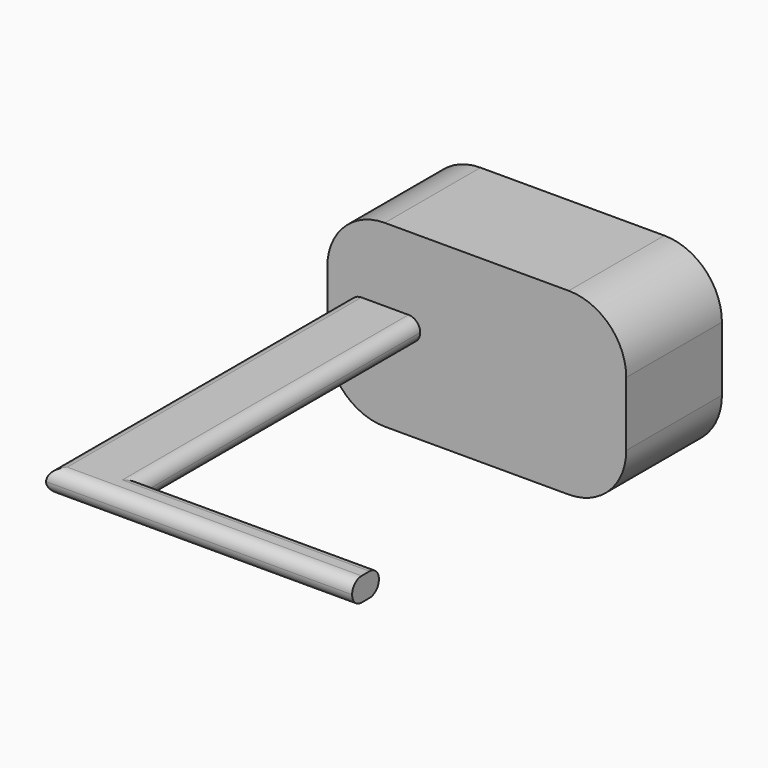
from build123d import *

# Parameters (mm, degrees)
F0_W     = 127
F0_H     = 76.2
F1_DEPTH = 50.8
F2_R     = 24.4421069165
F4_W     = 30
F4_H     = 10
F5_DEPTH = 211.9498550892
F6_W     = 14.2212212086
F6_H     = 10
F7_DEPTH = 100
F8_R     = 4.99999


# Not quite as in the source:
# - a fillet or chamfer is up to 0.001 mm smaller than in the source, because OpenCascade refuses the exact size


with BuildPart() as f1:
    # F0 (on Front) → F1 (new body)
    with BuildSketch(Plane.XZ):
        with Locations((21.6533541679, 32.7783897177)):
            Rectangle(F0_W, F0_H)
    extrude(amount=F1_DEPTH)

    # F2
    f2_edges = [f1.edges().sort_by_distance(p)[0] for p in [
        (-41.846646, -25.4, 70.87839),
        (-41.846646, -25.4, -5.32161),
        (85.153354, -25.4, -5.32161),
        (85.153354, -25.4, 70.87839),
    ]]
    fillet(f2_edges, radius=F2_R)

    # F4 (on face) → F5 (join)
    with BuildSketch(Plane(origin=(0, 0, 0), x_dir=(-1, 0, 0), z_dir=(0, 1, 0))):
        with Locations((17.3587081618, 34.757822752)):
            Rectangle(F4_W, F4_H)
    extrude(amount=-F5_DEPTH)

    # F6 (on face) → F7 (join)
    with BuildSketch(Plane.YZ.offset(-2.3587081618)):
        with Locations((-204.8392444849, 34.757822752)):
            Rectangle(F6_W, F6_H)
    extrude(amount=F7_DEPTH)

    # F8 (radius 5 in the source; OpenCascade refuses exactly that, so slightly less here)
    f8_edges = [f1.edges().sort_by_distance(p)[0] for p in [
        (-32.358708, -131.374928, 39.757823),
        (-32.358708, -131.374928, 29.757823),
        (32.641292, -211.949855, 29.757823),
        (-2.358708, -124.264317, 29.757823),
        (-2.358708, -124.264317, 39.757823),
        (47.641292, -197.728634, 39.757823),
        (32.641292, -211.949855, 39.757823),
        (47.641292, -197.728634, 29.757823),
    ]]
    fillet(f8_edges, radius=F8_R)


solid = f1.part
